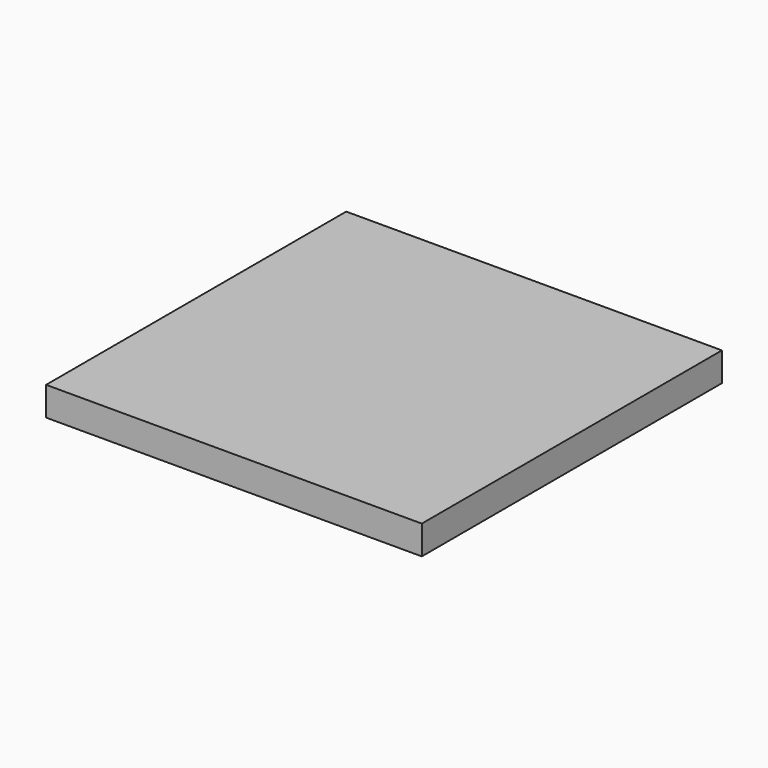
from build123d import *

# Parameters (mm, degrees)
F0_W     = 317.5
F0_H     = 25.4
F0_W_2   = 6.35
F1_DEPTH = 164.846


# Not quite as in the source:
# - ends of sketch curves that miss each other by under 0.0002 mm in the source are joined


with BuildPart() as f1:
    # F0 (on Front) → F1 (new body, symmetric)
    with BuildSketch(Plane.XZ):
        Rectangle(F0_W, F0_H)
        Polygon((165.1, 12.7), (158.75, 12.7), (158.75, -12.7), (165.1, -12.6999953677), align=None)
        with Locations((-161.925, 0)):
            Rectangle(F0_W_2, F0_H)
    extrude(amount=F1_DEPTH, both=True)


solid = f1.part
